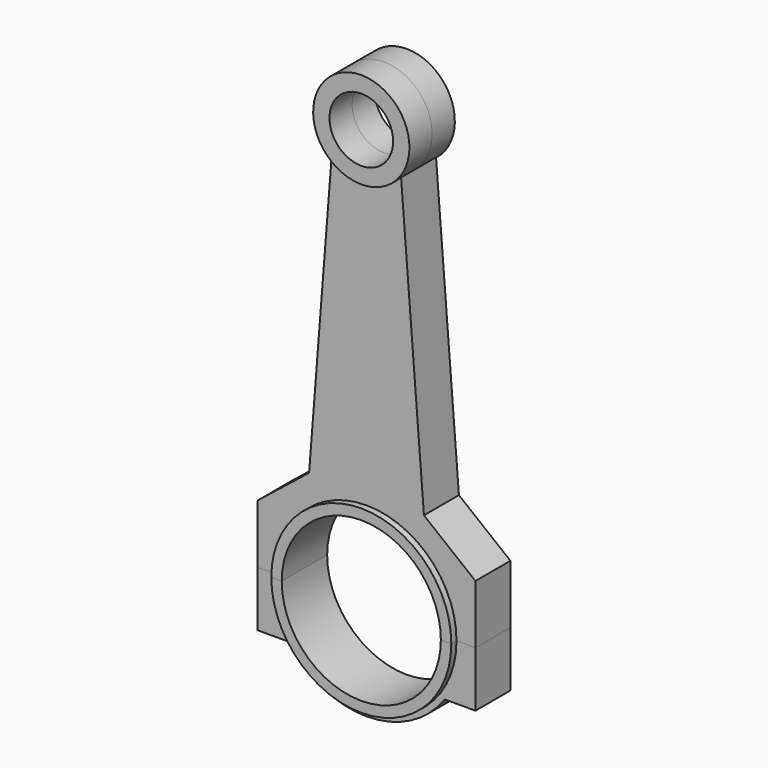
from build123d import *

# Parameters (mm, degrees)
F1_DEPTH = 11.049
F2_DEPTH = 11.049
F3_DEPTH = 8.509
F0_R     = 12.3825
F4_DEPTH = 11.049
F5_DEPTH = 8.509


with BuildPart() as f1:
    # F0 (on Front) → F1 (new body, symmetric)
    with BuildSketch(Plane.XZ):
        with BuildLine():
            ThreePointArc((-30.9626, 0), (0, 30.9626), (30.9626, 0))
            Line((30.9626, 0), (35.0266, 0))
            ThreePointArc((35.0266, 0), (0, 35.0266), (-35.0266, 0))
            Line((-35.0266, 0), (-30.9626, 0))
        make_face()
    extrude(amount=F1_DEPTH, both=True)

    # F0 (on Front) → F3 (join, symmetric)
    with BuildSketch(Plane.XZ):
        with BuildLine():
            ThreePointArc((-35.0266, 0), (0, 35.0266), (35.0266, 0))
            Line((35.0266, 0), (42.3926, 0))
            Line((42.3926, 0), (42.3926, 22.8854))
            Line((42.3926, 22.8854), (22.352, 38.862))
            Line((22.352, 38.862), (13.4496324754, 151.7054605291))
            ThreePointArc((13.4496324754, 151.7054605291), (0, 146.0119), (-13.4496324754, 151.7054605291))
            Line((-13.4496324754, 151.7054605291), (-22.352, 38.862))
            Line((-22.352, 38.862), (-42.3926, 22.8854))
            Line((-42.3926, 22.8854), (-42.3926, 0))
            Line((-42.3926, 0), (-35.0266, 0))
        make_face()
    extrude(amount=F3_DEPTH, both=True)

    # F0 (on Front) → F4 (join, symmetric)
    with BuildSketch(Plane.XZ):
        with BuildLine():
            ThreePointArc((-13.4496324754, 151.7054605291), (0, 146.0119), (13.4496324754, 151.7054605291))
            ThreePointArc((13.4496324754, 151.7054605291), (17.361621419, 157.710151074), (18.7325, 164.7444))
            ThreePointArc((18.7325, 164.7444), (-7.034248926, 182.106021419), (-13.4496324754, 151.7054605291))
        make_face()
        with Locations((0, 164.7444)):
            Circle(F0_R, mode=Mode.SUBTRACT)
    extrude(amount=F4_DEPTH, both=True)


with BuildPart() as f2:
    # F0 (on Front) → F2 (new body, symmetric)
    with BuildSketch(Plane.XZ):
        with BuildLine():
            Line((35.0266, 0), (30.9626, 0))
            ThreePointArc((30.9626, 0), (0, -30.9626), (-30.9626, 0))
            Line((-30.9626, 0), (-35.0266, 0))
            ThreePointArc((-35.0266, 0), (0, -35.0266), (35.0266, 0))
        make_face()
    extrude(amount=F2_DEPTH, both=True)

    # F0 (on Front) → F5 (join, symmetric)
    with BuildSketch(Plane.XZ):
        with BuildLine():
            Line((42.3926, 0), (35.0266, 0))
            ThreePointArc((35.0266, 0), (0, -35.0266), (-35.0266, 0))
            Line((-35.0266, 0), (-42.3926, 0))
            Line((-42.3926, 0), (-42.3926, -21.580753848))
            Line((-42.3926, -21.580753848), (-30.4384819285, -21.580753848))
            ThreePointArc((-30.4384819285, -21.580753848), (0, -37.3126), (30.4384819285, -21.580753848))
            Line((30.4384819285, -21.580753848), (42.3926, -21.580753848))
            Line((42.3926, -21.580753848), (42.3926, 0))
        make_face()
    extrude(amount=F5_DEPTH, both=True)


solid = Compound([f1.part, f2.part])
